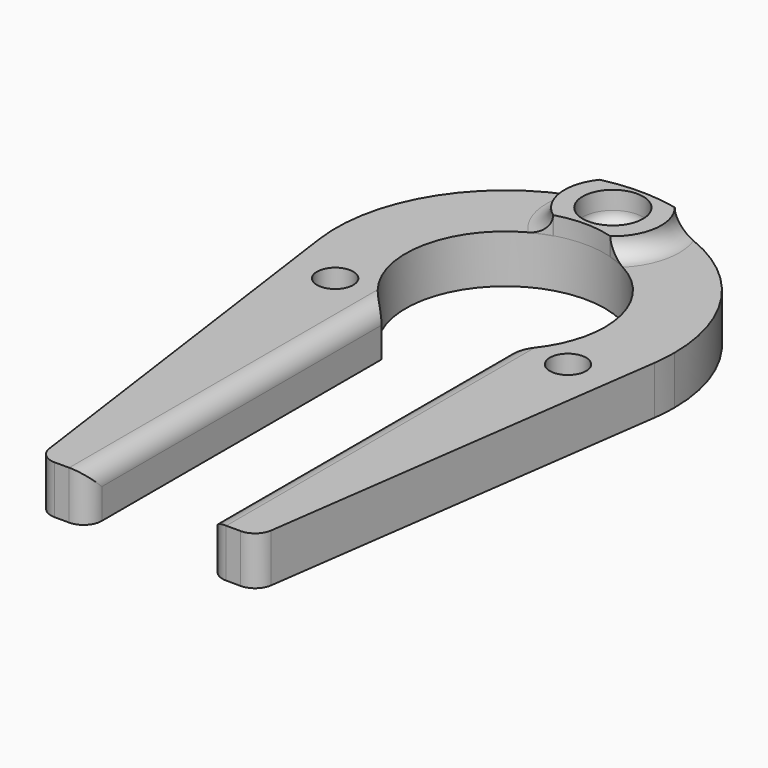
from build123d import *

# Parameters (mm, degrees)
F0_R         = 1.5
F1_DEPTH     = 4
F2_R         = 2.5
F2_R_2       = 1.5
F3_DEPTH     = 1.5
F4_R         = 2.5
F5_DEPTH     = 2.5
F6_R         = 0.99999
F7_T4_ANGLE  = 135.8501025958
F7_S5_R      = 8.25
F7_T6_DEPTH  = 9
F7_S7_R      = 14
F7_T8_DEPTH  = 9
F7_T12_ANGLE = 135.8501025958
F7_S13_R     = 8.25
F7_T14_DEPTH = 9
F7_S15_R     = 14
F7_T16_DEPTH = 9
F7_T17_DEPTH = 33.4377976258
F7_T19_DEPTH = 6.6124624953
F7_T21_DEPTH = 7


# Not quite as in the source:
# - a fillet or chamfer that OpenCascade refuses, or shapes differently, is made with other operations: its cross-section is extruded or revolved along the edge and cut away or added
# - a fillet or chamfer is up to 0.001 mm smaller than in the source, because OpenCascade refuses the exact size


with BuildPart() as f1:
    # F0 (on Top) → F1 (new body)
    with BuildSketch(Plane.XY):
        with BuildLine():
            ThreePointArc((-5, -6.5622023742), (-3.661454629, 7.3929865413), (8.25, 0))
            ThreePointArc((8.25, 0), (7.3929865413, -3.661454629), (5, -6.5622023742))
            Line((5, -6.5622023742), (5, -13.0766968306))
            ThreePointArc((5, -13.0766968306), (10.9584066623, -8.7128252263), (13.8671342987, -1.924210576))
            ThreePointArc((13.8671342987, -1.924210576), (13.9667440762, -0.9643961369), (14, 0))
            ThreePointArc((14, 0), (-0.9643961369, 13.9667440762), (-13.8671342987, -1.924210576))
            ThreePointArc((-13.8671342987, -1.924210576), (-10.9584066623, -8.7128252263), (-5, -13.0766968306))
            Line((-5, -13.0766968306), (-5, -6.5622023742))
        make_face()
        with Locations((-9.6345326171, -5.5625)):
            Circle(F0_R, mode=Mode.SUBTRACT)
        with Locations((9.6345326171, -5.5625)):
            Circle(F0_R, mode=Mode.SUBTRACT)
        with Locations((0, 11.125)):
            Circle(F0_R, mode=Mode.SUBTRACT)
        with BuildLine():
            Line((-5, -37), (-5, -13.0766968306))
            ThreePointArc((-5, -13.0766968306), (-10.9584066623, -8.7128252263), (-13.8671342987, -1.924210576))
            Line((-13.8671342987, -1.924210576), (-9, -37))
            Line((-9, -37), (-5, -37))
        make_face()
        with BuildLine():
            ThreePointArc((13.8671342987, -1.924210576), (10.9584066623, -8.7128252263), (5, -13.0766968306))
            Line((5, -13.0766968306), (5, -37))
            Line((5, -37), (9, -37))
            Line((9, -37), (13.8671342987, -1.924210576))
        make_face()
    extrude(amount=F1_DEPTH)

    # F2 (on face) → F3 (join)
    with BuildSketch(Plane.XY.offset(4)):
        with BuildLine():
            ThreePointArc((4, 11.125), (3.7683876751, 12.466362863), (3.1003728348, 13.6523876404))
            ThreePointArc((3.1003728348, 13.6523876404), (0, 14), (-3.1003728348, 13.6523876404))
            ThreePointArc((-3.1003728348, 13.6523876404), (-3.9680776614, 10.6206591696), (-2.3695505017, 7.9023876404))
            ThreePointArc((-2.3695505017, 7.9023876404), (0, 8.25), (2.3695505017, 7.9023876404))
            ThreePointArc((2.3695505017, 7.9023876404), (3.5691877232, 9.3192040545), (4, 11.125))
        make_face()
        with Locations((0, 11.125)):
            Circle(F2_R, mode=Mode.SUBTRACT)
        with Locations((0, 11.125)):
            Circle(F2_R)
        with Locations((0, 11.125)):
            Circle(F2_R_2, mode=Mode.SUBTRACT)
        with Locations((0, 11.125)):
            Circle(F2_R_2)
    extrude(amount=F3_DEPTH)

    # F4 (on face) → F5 (cut)
    with BuildSketch(Plane.XY.offset(5.5)):
        with Locations((0, 11.125)):
            Circle(F4_R)
    extrude(amount=-F5_DEPTH, mode=Mode.SUBTRACT)

    # F6 (radius 1 in the source; OpenCascade refuses exactly that, so slightly less here)
    f6_edges = [f1.edges().sort_by_distance(p)[0] for p in [
        (-2.5, 11.125, 3),
    ]]
    fillet(f6_edges, radius=F6_R)

    # F7: fillet of radius 1.5 on 8 edges, made by hand


with BuildPart() as f7_tool2:
    # F7_s3 → F7_t4 (revolve)
    with BuildSketch(Plane(origin=(4.7497345288, 2.6674303712, 0), x_dir=(0, 0, 1), z_dir=(0.8719122535, 0.489662151, 0))):
        with BuildLine():
            ThreePointArc((5.5, -13.7000238206), (4.4393398282, -14.1393636488), (4, -15.2000238206))
            Line((4, -15.2000238206), (3.97, -15.2000238206))
            Line((3.97, -15.2000238206), (3.97, -13.6700238206))
            Line((3.97, -13.6700238206), (5.5, -13.6700238206))
            Line((5.5, -13.6700238206), (5.5, -13.7000238206))
        make_face()
    revolve(axis=Axis((0, 11.125, 4), (0, 0, 1)), revolution_arc=F7_T4_ANGLE)

    # F7_s5 → F7_t6 (cut, symmetric)
    with BuildSketch(Plane.XY.offset(4.7)):
        Circle(F7_S5_R)
    extrude(amount=F7_T6_DEPTH, both=True, mode=Mode.SUBTRACT)

    # F7_s7 → F7_t8 (intersect, symmetric)
    with BuildSketch(Plane.XY.offset(4.7)):
        Circle(F7_S7_R)
    extrude(amount=F7_T8_DEPTH, both=True, mode=Mode.INTERSECT)


with BuildPart() as f1_1:
    add(f1.part)

    # F7_t1: union F7_tool2
    add(f7_tool2.part)


with BuildPart() as f7_tool10:
    # F7_s11 → F7_t12 (revolve)
    with BuildSketch(Plane(origin=(2.7528712992, 0.7289603177, 0), x_dir=(0, 0, 1), z_dir=(-0.9666827179, -0.2559775829, 0))):
        with BuildLine():
            ThreePointArc((5.5, 6.7543452365), (4.4393398282, 6.3150054083), (4, 5.2543452365))
            Line((4, 5.2543452365), (3.97, 5.2543452365))
            Line((3.97, 5.2543452365), (3.97, 6.7843452365))
            Line((3.97, 6.7843452365), (5.5, 6.7843452365))
            Line((5.5, 6.7843452365), (5.5, 6.7543452365))
        make_face()
    revolve(axis=Axis((0, 11.125, 4), (0, 0, 1)), revolution_arc=F7_T12_ANGLE)

    # F7_s13 → F7_t14 (cut, symmetric)
    with BuildSketch(Plane.XY.offset(5.3)):
        Circle(F7_S13_R)
    extrude(amount=F7_T14_DEPTH, both=True, mode=Mode.SUBTRACT)

    # F7_s15 → F7_t16 (intersect, symmetric)
    with BuildSketch(Plane.XY.offset(5.3)):
        Circle(F7_S15_R)
    extrude(amount=F7_T16_DEPTH, both=True, mode=Mode.INTERSECT)


with BuildPart() as f1_2:
    add(f1_1.part)

    # F7_t9: union F7_tool10
    add(f7_tool10.part)

    # F7_s18 → F7_t17 (cut)
    with BuildSketch(Plane.XZ.offset(5.0622023742)):
        with BuildLine():
            ThreePointArc((6.5, 4), (5.4393398282, 3.5606601718), (5, 2.5))
            Line((5, 2.5), (4.97, 2.5))
            Line((4.97, 2.5), (4.97, 4.03))
            Line((4.97, 4.03), (6.5, 4.03))
            Line((6.5, 4.03), (6.5, 4))
        make_face()
        with BuildLine():
            ThreePointArc((-5, 2.5), (-5.4393398282, 3.5606601718), (-6.5, 4))
            Line((-6.5, 4), (-6.5, 4.03))
            Line((-6.5, 4.03), (-4.97, 4.03))
            Line((-4.97, 4.03), (-4.97, 2.5))
            Line((-4.97, 2.5), (-5, 2.5))
        make_face()
    extrude(amount=F7_T17_DEPTH, mode=Mode.SUBTRACT)

    # F7_s20 → F7_t19 (cut)
    with BuildSketch(Plane.XY.offset(-1.3062312476)):
        with BuildLine():
            ThreePointArc((-9.1795331415, -35.7061654189), (-8.6788453666, -36.631204696), (-7.6937687524, -37))
            Line((-7.6937687524, -37), (-7.6937687524, -37.03))
            Line((-7.6937687524, -37.03), (-9.026124625, -37.03))
            Line((-9.026124625, -37.03), (-9.2092484293, -35.7102887272))
            Line((-9.2092484293, -35.7102887272), (-9.1795331415, -35.7061654189))
        make_face()
        with BuildLine():
            ThreePointArc((7.6937687524, -37), (8.6788453666, -36.631204696), (9.1795331415, -35.7061654189))
            Line((9.1795331415, -35.7061654189), (9.2092484293, -35.7102887272))
            Line((9.2092484293, -35.7102887272), (9.026124625, -37.03))
            Line((9.026124625, -37.03), (7.6937687524, -37.03))
            Line((7.6937687524, -37.03), (7.6937687524, -37))
        make_face()
    extrude(amount=F7_T19_DEPTH, mode=Mode.SUBTRACT)

    # F7_s22 → F7_t21 (cut)
    with BuildSketch(Plane.XY.offset(-1.5)):
        with BuildLine():
            ThreePointArc((5, -35.5), (5.4393398282, -36.5606601718), (6.5, -37))
            Line((6.5, -37), (6.5, -37.03))
            Line((6.5, -37.03), (4.97, -37.03))
            Line((4.97, -37.03), (4.97, -35.5))
            Line((4.97, -35.5), (5, -35.5))
        make_face()
        with BuildLine():
            ThreePointArc((-6.5, -37), (-5.4393398282, -36.5606601718), (-5, -35.5))
            Line((-5, -35.5), (-4.97, -35.5))
            Line((-4.97, -35.5), (-4.97, -37.03))
            Line((-4.97, -37.03), (-6.5, -37.03))
            Line((-6.5, -37.03), (-6.5, -37))
        make_face()
    extrude(amount=F7_T21_DEPTH, mode=Mode.SUBTRACT)


solid = f1_2.part
